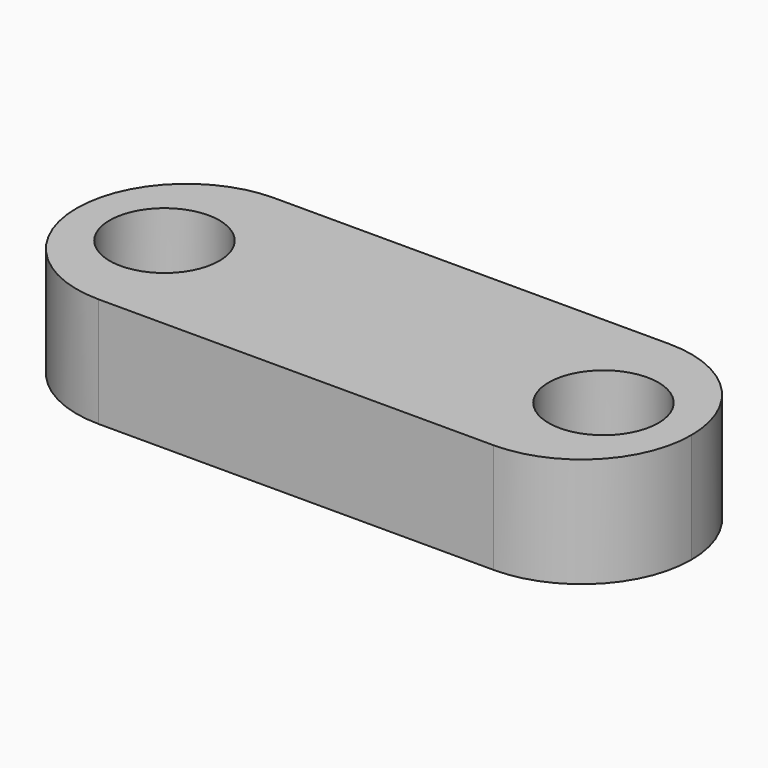
from build123d import *

# Parameters (mm, degrees)
F0_W     = 56
F0_H     = 20
F0_R     = 5
F1_DEPTH = 10
F2_R     = 9.99999


# Not quite as in the source:
# - a fillet or chamfer is up to 0.001 mm smaller than in the source, because OpenCascade refuses the exact size


with BuildPart() as f1:
    # F0 (on Top) → F1 (new body)
    with BuildSketch(Plane.XY):
        Rectangle(F0_W, F0_H)
        with Locations((-20, 0)):
            Circle(F0_R, mode=Mode.SUBTRACT)
        with Locations((20, 0)):
            Circle(F0_R, mode=Mode.SUBTRACT)
    extrude(amount=F1_DEPTH)

    # F2 (radius 10 in the source; OpenCascade refuses exactly that, so slightly less here)
    f2_edges = [f1.edges().sort_by_distance(p)[0] for p in [
        (-28, 10, 5),
        (-28, -10, 5),
        (28, 10, 5),
        (28, -10, 5),
    ]]
    fillet(f2_edges, radius=F2_R)


solid = f1.part
